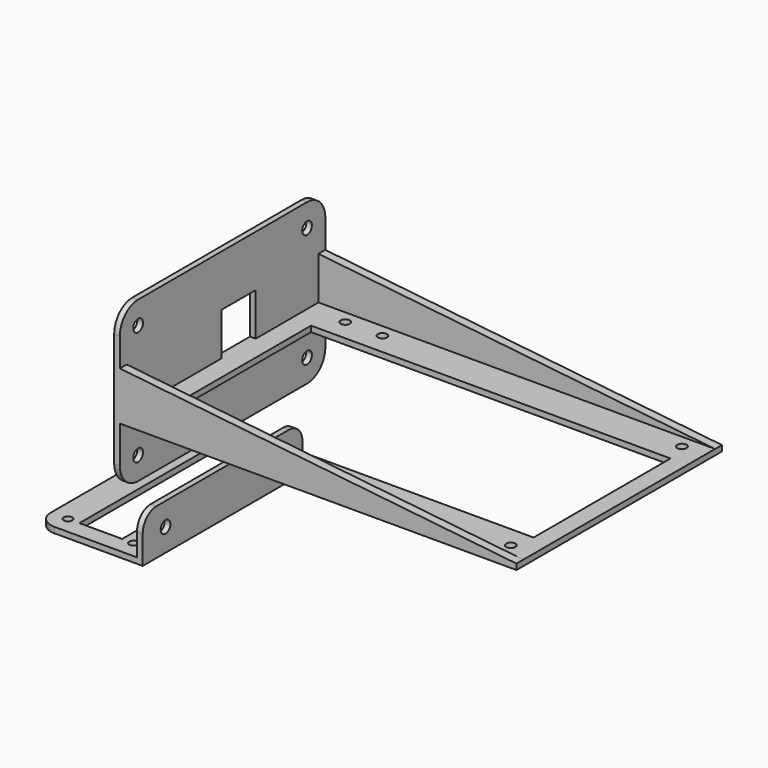
from build123d import *

# Parameters (mm, degrees)
F0_W       = 1
F0_H       = 90
F0_R       = 1.625
F0_W_2     = 126
F0_H_2     = 60
F1_DEPTH   = 2
F2_R       = 2.125
F2_W       = 90
F2_H       = 21
F3_DEPTH   = 2
F4_R       = 8
F5_W       = 3
F5_H       = 15
F6_DEPTH   = 139
F7_SIZE2   = 14.99999
F7_SIZE    = 138.99999
F7_2_SIZE2 = 14.99999
F7_2_SIZE  = 138.99999
F9_W       = 35
F9_H       = 70
F9_R       = 1.5
F9_W_2     = 15
F9_H_2     = 58
F10_DEPTH  = 2
F11_W      = 70
F11_H      = 14
F11_R      = 2.125
F11_H_2    = 2
F12_DEPTH  = 2
F13_R      = 6


# Not quite as in the source:
# - a fillet or chamfer is up to 0.001 mm smaller than in the source, because OpenCascade refuses the exact size
# - a feature names something its author has since deleted; it is built from what else it names


with BuildPart() as f1:
    # F0 (on Top) → F1 (new body)
    with BuildSketch(Plane.XY):
        with Locations((-70.5, -45)):
            Rectangle(F0_W, F0_H)
        Polygon((0, 0), (-70, 0), (-70, -90), (68, -90), (68, 0), align=None)
        with Locations((-58, -82.5)):
            Circle(F0_R, mode=Mode.SUBTRACT)
        with Locations((60, -82.5)):
            Circle(F0_R, mode=Mode.SUBTRACT)
        with Locations((-1, -45)):
            Rectangle(F0_W_2, F0_H_2, mode=Mode.SUBTRACT)
        with Locations((-58, -7.5)):
            Circle(F0_R, mode=Mode.SUBTRACT)
        with Locations((-45, -7.5)):
            Circle(F0_R, mode=Mode.SUBTRACT)
        with Locations((60, -7.5)):
            Circle(F0_R, mode=Mode.SUBTRACT)
    extrude(amount=-F1_DEPTH)

    # F2 (on face) → F3 (join)
    with BuildSketch(Plane(origin=(-71, 0, 0), x_dir=(0, -1, 0), z_dir=(-1, 0, 0))):
        Polygon((90, 33), (0, 33), (0, 0), (30.5, 0), (30.5, 15), (45.5, 15), (45.5, 0), (90, 0), align=None)
        with Locations((8, 25)):
            Circle(F2_R, mode=Mode.SUBTRACT)
        with Locations((82, 25)):
            Circle(F2_R, mode=Mode.SUBTRACT)
        with Locations((45, -12.5)):
            Rectangle(F2_W, F2_H)
        with Locations((8, -15)):
            Circle(F2_R, mode=Mode.SUBTRACT)
        with Locations((82, -15)):
            Circle(F2_R, mode=Mode.SUBTRACT)
        Polygon((30.5, 0), (0, 0), (0, -2), (90, -2), (90, 0), (45.5, 0), align=None)
    extrude(amount=F3_DEPTH)

    # F4
    f4_edges = [f1.edges().sort_by_distance(p)[0] for p in [
        (-72, -90, 33),
        (-72, -90, -23),
        (-72, 0, -23),
        (-72, 0, 33),
    ]]
    fillet(f4_edges, radius=F4_R)

    # F5 (on face) → F6 (join)
    with BuildSketch(Plane(origin=(-71, 0, 0), x_dir=(0, -1, 0), z_dir=(-1, 0, 0))):
        with Locations((88.5, 7.5)):
            Rectangle(F5_W, F5_H)
        with Locations((1.5, 7.5)):
            Rectangle(F5_W, F5_H)
    extrude(amount=-F6_DEPTH)

    # F7 (size 139 and 15 in the source; OpenCascade refuses exactly that, so slightly less here)
    f7_edges = [f1.edges().sort_by_distance(p)[0] for p in [
        (68, -88.5, 15),
    ]]
    f7_side = f1.faces().sort_by_distance((-1.5, -88.5, 15))[0]
    chamfer(f7_edges, length=F7_SIZE, length2=F7_SIZE2, reference=f7_side)

    # F7#2 (size 139 and 15 in the source; OpenCascade refuses exactly that, so slightly less here)
    f7_2_edges = [f1.edges().sort_by_distance(p)[0] for p in [
        (68, -1.5, 15),
    ]]
    f7_2_side = f1.faces().sort_by_distance((-1.5, -1.5, 15))[0]
    chamfer(f7_2_edges, length=F7_2_SIZE, length2=F7_2_SIZE2, reference=f7_2_side)


with BuildPart() as f10:
    # F9 (on offset) → F10 (new body)
    with BuildSketch(Plane.XY.offset(-50)):
        with Locations((-90.5, -45)):
            Rectangle(F9_W, F9_H)
        with Locations((-102, -74)):
            Circle(F9_R, mode=Mode.SUBTRACT)
        with Locations((-79, -74)):
            Circle(F9_R, mode=Mode.SUBTRACT)
        with Locations((-102, -16)):
            Circle(F9_R, mode=Mode.SUBTRACT)
        with Locations((-90.5, -45)):
            Rectangle(F9_W_2, F9_H_2, mode=Mode.SUBTRACT)
        with Locations((-79, -16)):
            Circle(F9_R, mode=Mode.SUBTRACT)
    extrude(amount=F10_DEPTH)

    # F11 (on face) → F12 (join)
    with BuildSketch(Plane.YZ.offset(-73)):
        with Locations((-45, -41)):
            Rectangle(F11_W, F11_H)
        with Locations((-70, -42)):
            Circle(F11_R, mode=Mode.SUBTRACT)
        with Locations((-20, -42)):
            Circle(F11_R, mode=Mode.SUBTRACT)
        with Locations((-45, -49)):
            Rectangle(F11_W, F11_H_2)
    extrude(amount=F12_DEPTH)

    # F13
    f13_edges = [f10.edges().sort_by_distance(p)[0] for p in [
        (-108, -10, -49),
        (-108, -80, -49),
        (-72, -80, -34),
        (-72, -10, -34),
    ]]
    fillet(f13_edges, radius=F13_R)


solid = Compound([f1.part, f10.part])
